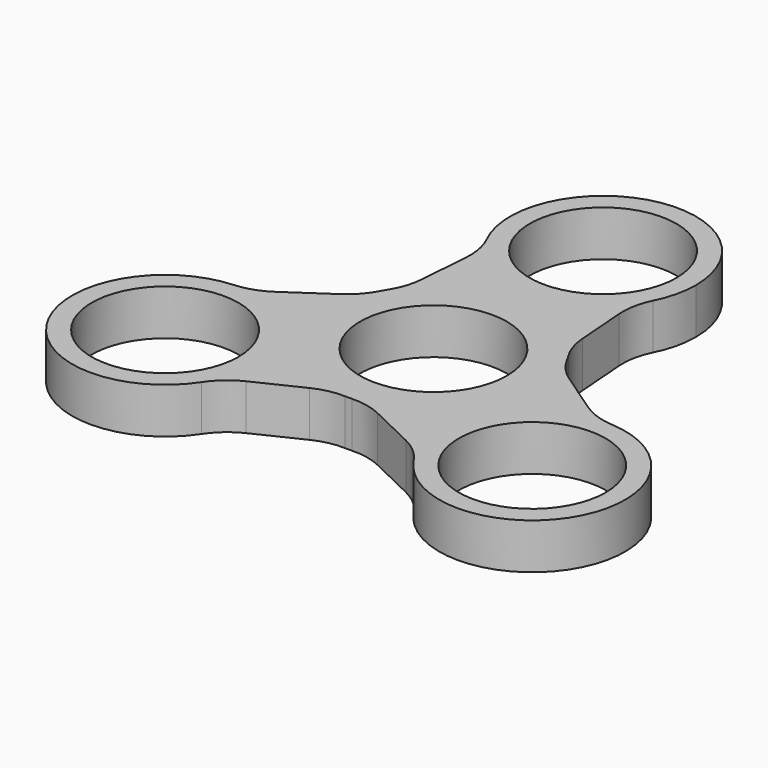
from build123d import *

# Parameters (mm, degrees)
F0_R     = 11.25
F1_DEPTH = 7
F2_R     = 10


# Not quite as in the source:
# - a feature names something its author has since deleted; it is built from what else it names


with BuildPart() as f1:
    # F0 (on Top) → F1 (new body)
    with BuildSketch(Plane.XY):
        with BuildLine():
            ThreePointArc((2.7119035956, -16.0221121856), (12.4123110948, -10.4879470482), (16.25, 0))
            ThreePointArc((16.25, 0), (15.9933502519, 2.8766730299), (15.2315079728, 5.6624786864))
            ThreePointArc((15.2315079728, 5.6624786864), (14.0729128115, 8.125), (12.5196043772, 10.3596334992))
            ThreePointArc((12.5196043772, 10.3596334992), (0, 16.25), (-12.5196043772, 10.3596334992))
            ThreePointArc((-12.5196043772, 10.3596334992), (-14.0729128115, 8.125), (-15.2315079728, 5.6624786864))
            ThreePointArc((-15.2315079728, 5.6624786864), (-14.0729128115, -8.125), (-2.7119035956, -16.0221121856))
            ThreePointArc((-2.7119035956, -16.0221121856), (0, -16.25), (2.7119035956, -16.0221121856))
        make_face()
        Circle(F0_R, mode=Mode.SUBTRACT)
        with BuildLine():
            ThreePointArc((15.2315079728, 5.6624786864), (15.9933502519, 2.8766730299), (16.25, 0))
            ThreePointArc((16.25, 0), (12.4123110948, -10.4879470482), (2.7119035956, -16.0221121856))
            Line((2.7119035956, -16.0221121856), (15.101342571, -21.9861975129))
            ThreePointArc((15.101342571, -21.9861975129), (15.8049636191, -9.125), (26.5912768643, -2.0850475413))
            Line((26.5912768643, -2.0850475413), (15.2315079728, 5.6624786864))
        make_face()
        with BuildLine():
            ThreePointArc((-12.5196043772, 10.3596334992), (0, 16.25), (12.5196043772, 10.3596334992))
            Line((12.5196043772, 10.3596334992), (11.4899342932, 24.0712450542))
            ThreePointArc((11.4899342932, 24.0712450542), (0, 18.25), (-11.4899342932, 24.0712450542))
            Line((-11.4899342932, 24.0712450542), (-12.5196043772, 10.3596334992))
        make_face()
        with BuildLine():
            ThreePointArc((42.395825623, -16.25), (37.6566137131, -5.6383361387), (26.5912768643, -2.0850475413))
            ThreePointArc((26.5912768643, -2.0850475413), (15.8049636191, -9.125), (15.101342571, -21.9861975129))
            ThreePointArc((15.101342571, -21.9861975129), (31.0765777883, -30.1953645254), (42.395825623, -16.25))
        make_face()
        with Locations((28.145825623, -16.25)):
            Circle(F0_R, mode=Mode.SUBTRACT)
        with BuildLine():
            Line((-15.101342571, -21.9861975129), (-2.7119035956, -16.0221121856))
            ThreePointArc((-2.7119035956, -16.0221121856), (-14.0729128115, -8.125), (-15.2315079728, 5.6624786864))
            Line((-15.2315079728, 5.6624786864), (-26.5912768643, -2.0850475413))
            ThreePointArc((-26.5912768643, -2.0850475413), (-17.5341617617, -6.7392119099), (-13.895825623, -16.25))
            ThreePointArc((-13.895825623, -16.25), (-14.2004610976, -19.1807521653), (-15.101342571, -21.9861975129))
        make_face()
        with BuildLine():
            ThreePointArc((-11.4899342932, 24.0712450542), (0, 18.25), (11.4899342932, 24.0712450542))
            ThreePointArc((11.4899342932, 24.0712450542), (13.5424160267, 28.0654235647), (14.25, 32.5))
            ThreePointArc((14.25, 32.5), (-4.4345764353, 46.0424160267), (-11.4899342932, 24.0712450542))
        make_face()
        with Locations((0, 32.5)):
            Circle(F0_R, mode=Mode.SUBTRACT)
        with BuildLine():
            ThreePointArc((-26.5912768643, -2.0850475413), (-40.4866876269, -23.375), (-15.101342571, -21.9861975129))
            ThreePointArc((-15.101342571, -21.9861975129), (-14.2004610976, -19.1807521653), (-13.895825623, -16.25))
            ThreePointArc((-13.895825623, -16.25), (-17.5341617617, -6.7392119099), (-26.5912768643, -2.0850475413))
        make_face()
        with Locations((-28.145825623, -16.25)):
            Circle(F0_R, mode=Mode.SUBTRACT)
    extrude(amount=F1_DEPTH)

    # F2
    f2_edges = [f1.edges().sort_by_distance(p)[0] for p in [
        (-11.489934, 24.071245, 3.5),
        (-12.519604, 10.359633, 3.5),
        (-15.231508, 5.662479, 3.5),
        (-26.591277, -2.085048, 3.5),
        (2.711904, -16.022112, 3.5),
        (-2.711904, -16.022112, 3.5),
        (15.101343, -21.986198, 3.5),
        (-15.101343, -21.986198, 3.5),
        (26.591277, -2.085048, 3.5),
        (15.231508, 5.662479, 3.5),
        (12.519604, 10.359633, 3.5),
        (11.489934, 24.071245, 3.5),
    ]]
    fillet(f2_edges, radius=F2_R)


solid = f1.part
